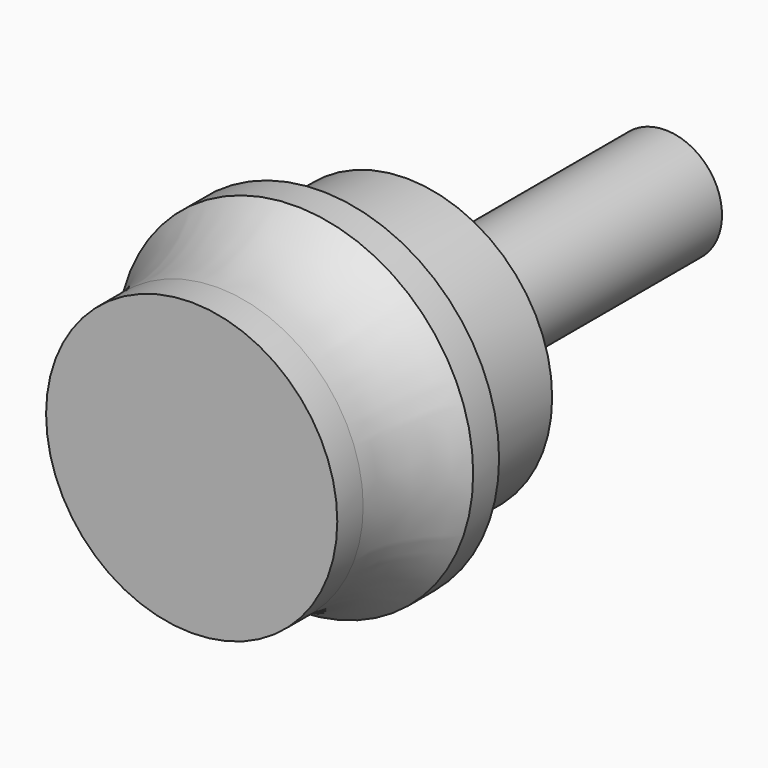
from build123d import *

# Parameters (mm, degrees)
F0_R     = 4.5
F1_DEPTH = 5
F2_DEPTH = 3.3
F3_R     = 5.5
F4_DEPTH = 1
F6_R     = 1.75
F7_DEPTH = 10


# Not quite as in the source:
# - a fillet or chamfer that OpenCascade refuses, or shapes differently, is made with other operations: its cross-section is extruded or revolved along the edge and cut away or added


with BuildPart() as f1:
    # F0 (on Front) → F1 (new body)
    with BuildSketch(Plane.XZ):
        Circle(F0_R)
    extrude(amount=F1_DEPTH)

    # F2 (add): a face of the model
    f2_faces = [f1.faces().sort_by_distance(p)[0] for p in [
        (0, 0, 0),
    ]]
    extrude(f2_faces, amount=F2_DEPTH)

    # F3 (on Front) → F4 (join)
    with BuildSketch(Plane.XZ):
        Circle(F3_R)
    extrude(amount=F4_DEPTH)

    # F5: fillet of radius 5 on 1 edges, made by hand

    # F5_s1 → F5_t2 (revolve)
    with BuildSketch(Plane.XY):
        with BuildLine():
            ThreePointArc((5.5, -1), (4.7565835097, -2.4188611699), (4.5, -4))
            Line((4.5, -4), (4.5, -1))
            Line((4.5, -1), (5.5, -1))
        make_face()
    revolve(axis=Axis((0, -1, 0), (0, 1, 0)))

    # F6 (on face) → F7 (join)
    with BuildSketch(Plane(origin=(0, 3.3, 0), x_dir=(-1, 0, 0), z_dir=(0, 1, 0))):
        Circle(F6_R)
    extrude(amount=F7_DEPTH)


solid = f1.part
